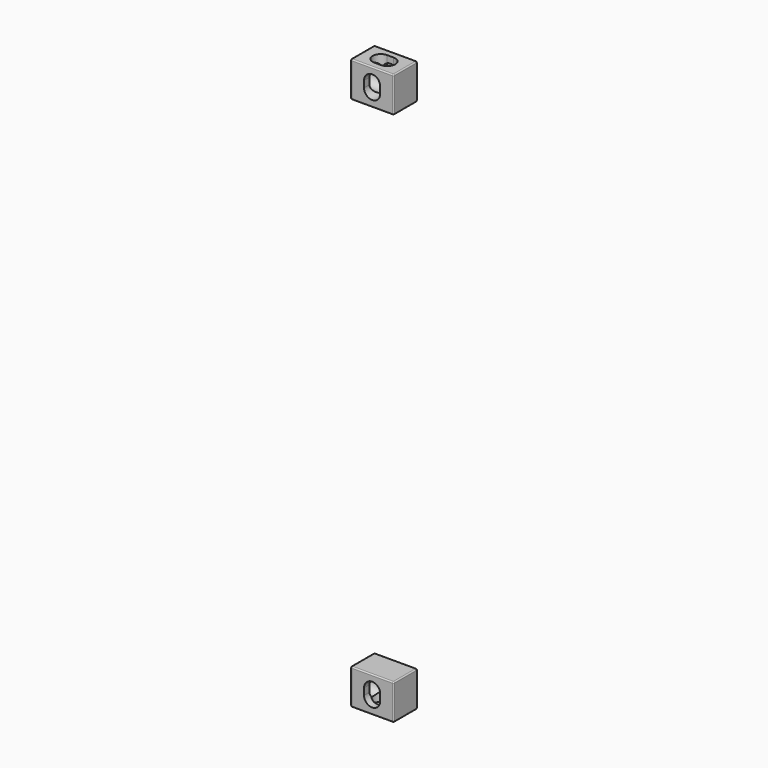
from build123d import *

# Parameters (mm, degrees)
F0_W          = 184
F0_H          = 127
F1_DEPTH      = 152
F3_DEPTH      = 122
F5_DEPTH      = 92
F7_DEPTH      = 78
F8_R          = 5
F9_R          = 5
F10_T1_DEPTH  = 159.5
F10_T3_DEPTH  = 142
F10_T5_DEPTH  = 191.5
F10_T7_DEPTH  = 117
F10_S11_W     = 5
F10_S11_H     = 5
F10_T12_DEPTH = 5
F10_S17_W     = 5
F10_S17_H     = 5
F10_T18_DEPTH = 5
F10_S23_W     = 5
F10_S23_H     = 5
F10_T24_DEPTH = 5
F10_S29_W     = 5
F10_S29_H     = 5
F10_T30_DEPTH = 5
F11_T1_DEPTH  = 117
F11_S5_W      = 5
F11_S5_H      = 5
F11_T6_DEPTH  = 5
F11_S11_W     = 5
F11_S11_H     = 5
F11_T12_DEPTH = 5


# Not quite as in the source:
# - a fillet or chamfer that OpenCascade refuses, or shapes differently, is made with other operations: its cross-section is extruded or revolved along the edge and cut away or added


with BuildPart() as f1:
    # F0 (on Top) → F1 (new body)
    with BuildSketch(Plane.XY):
        with Locations((-47.3488530219, 42.2096716464)):
            Rectangle(F0_W, F0_H)
    extrude(amount=F1_DEPTH)

    # F2 (on face) → F3 (cut)
    with BuildSketch(Plane.XZ.offset(21.2903283536)):
        with BuildLine():
            Line((-81.879962092, 90), (-81.879962092, 76))
            Line((-81.879962092, 76), (-81.879962092, 62))
            ThreePointArc((-81.879962092, 62), (-47.3488530219, 27.4688909298), (-12.8177439517, 62))
            Line((-12.8177439517, 62), (-12.8177439517, 76))
            Line((-12.8177439517, 76), (-12.8177439517, 90))
            ThreePointArc((-12.8177439517, 90), (-47.3488530219, 124.5311090702), (-81.879962092, 90))
        make_face()
    extrude(amount=-F3_DEPTH, mode=Mode.SUBTRACT)

    # F4 (on face) → F5 (cut)
    with BuildSketch(Plane(origin=(-139.3488530219, 0, 0), x_dir=(0, -1, 0), z_dir=(-1, 0, 0))):
        with BuildLine():
            Line((-76.7407790178, 90.0138813162), (-76.7407790178, 76.0138813162))
            Line((-76.7407790178, 76.0138813162), (-76.7407790178, 62.0138813162))
            ThreePointArc((-76.7407790178, 62.0138813162), (-42.2096699476, 27.482772246), (-7.6785608775, 62.0138813162))
            Line((-7.6785608775, 62.0138813162), (-7.6785608775, 76.0138813162))
            Line((-7.6785608775, 76.0138813162), (-7.6785608775, 90.0138813162))
            ThreePointArc((-7.6785608775, 90.0138813162), (-42.2096699476, 124.5449903863), (-76.7407790178, 90.0138813162))
        make_face()
    extrude(amount=-F5_DEPTH, mode=Mode.SUBTRACT)

    # F6 (on face) → F7 (cut)
    with BuildSketch(Plane.XY.offset(152)):
        with BuildLine():
            Line((-33.3898597658, 76.7718884866), (-47.3898597658, 76.7718884866))
            Line((-47.3898597658, 76.7718884866), (-61.3898597658, 76.7718884866))
            ThreePointArc((-61.3898597658, 76.7718884866), (-95.9209688359, 42.2407794164), (-61.3898597658, 7.7096703462))
            Line((-61.3898597658, 7.7096703462), (-47.3898597658, 7.7096703462))
            Line((-47.3898597658, 7.7096703462), (-33.3898597658, 7.7096703462))
            ThreePointArc((-33.3898597658, 7.7096703462), (1.1412493044, 42.2407794164), (-33.3898597658, 76.7718884866))
        make_face()
    extrude(amount=-F7_DEPTH, mode=Mode.SUBTRACT)

    # F8
    f8_edges = [f1.edges().sort_by_distance(p)[0] for p in [
        (-47.348853, -21.290328, 152),
    ]]
    fillet(f8_edges, radius=F8_R)

    # F9
    f9_edges = [f1.edges().sort_by_distance(p)[0] for p in [
        (-139.348853, -21.290328, 73.5),
        (-139.348853, 44.709672, 152),
        (44.651147, 44.709672, 152),
        (-47.348853, 105.709672, 152),
        (44.651147, -21.290328, 73.5),
        (-47.348853, -21.290328, 0),
    ]]
    fillet(f9_edges, radius=F9_R)

    # F10: fillet of radius 5 on 4 edges, made by hand

    # F10_s2 → F10_t1 (cut)
    with BuildSketch(Plane.XY.offset(-12.5)):
        with BuildLine():
            ThreePointArc((-134.3488530219, 105.7096716464), (-137.8843869278, 104.2452055523), (-139.3488530219, 100.7096716464))
            Line((-139.3488530219, 100.7096716464), (-139.3488530219, 105.7096716464))
            Line((-139.3488530219, 105.7096716464), (-134.3488530219, 105.7096716464))
        make_face()
    extrude(amount=F10_T1_DEPTH, mode=Mode.SUBTRACT)

    # F10_s4 → F10_t3 (cut)
    with BuildSketch(Plane.XY.offset(5)):
        with BuildLine():
            ThreePointArc((44.6511469781, 100.7096716464), (43.1866808841, 104.2452055523), (39.6511469781, 105.7096716464))
            Line((39.6511469781, 105.7096716464), (44.6511469781, 105.7096716464))
            Line((44.6511469781, 105.7096716464), (44.6511469781, 100.7096716464))
        make_face()
    extrude(amount=F10_T3_DEPTH, mode=Mode.SUBTRACT)

    # F10_s6 → F10_t5 (cut)
    with BuildSketch(Plane.YZ.offset(-151.8488530219)):
        with BuildLine():
            ThreePointArc((100.7096716464, 0), (104.2452055523, 1.4644660941), (105.7096716464, 5))
            Line((105.7096716464, 5), (105.7096716464, 0))
            Line((105.7096716464, 0), (100.7096716464, 0))
        make_face()
    extrude(amount=F10_T5_DEPTH, mode=Mode.SUBTRACT)

    # F10_s8 → F10_t7 (cut)
    with BuildSketch(Plane.XZ.offset(-100.7096716464)):
        with BuildLine():
            ThreePointArc((44.6511469781, 5), (43.1866808841, 1.4644660941), (39.6511469781, 0))
            Line((39.6511469781, 0), (44.6511469781, 0))
            Line((44.6511469781, 0), (44.6511469781, 5))
        make_face()
    extrude(amount=F10_T7_DEPTH, mode=Mode.SUBTRACT)


with BuildPart() as f10_tool10:
    # F10_s11 → F10_t12 (new body)
    with BuildSketch(Plane.YZ.offset(39.6511469781)):
        with Locations((-18.7903283536, 2.5)):
            Rectangle(F10_S11_W, F10_S11_H)
    extrude(amount=F10_T12_DEPTH)

    # F10_s13 → F10_t14 (revolve, cut)
    with BuildSketch(Plane(origin=(39.6511469781, -16.2903283536, 5), x_dir=(0, 0.7071067812, 0.7071067812), z_dir=(0, 0.7071067812, -0.7071067812))):
        with BuildLine():
            ThreePointArc((0, -5), (5, 0), (0, 5))
            Line((0, 5), (0, -5))
        make_face()
    revolve(axis=Axis((39.6511469781, -16.2903283536, 5), (1, 0, 0)), mode=Mode.SUBTRACT)


with BuildPart() as f1_1:
    add(f1.part)

    # F10_t9: cut F10_tool10
    add(f10_tool10.part, mode=Mode.SUBTRACT)


with BuildPart() as f10_tool16:
    # F10_s17 → F10_t18 (new body)
    with BuildSketch(Plane.YZ.offset(39.6511469781)):
        with Locations((103.2096716464, 149.5)):
            Rectangle(F10_S17_W, F10_S17_H)
    extrude(amount=F10_T18_DEPTH)

    # F10_s19 → F10_t20 (revolve, cut)
    with BuildSketch(Plane(origin=(39.6511469781, 100.7096716464, 147), x_dir=(0, -0.7071067812, -0.7071067812), z_dir=(0, -0.7071067812, 0.7071067812))):
        with BuildLine():
            ThreePointArc((0, -5), (5, 0), (0, 5))
            Line((0, 5), (0, -5))
        make_face()
    revolve(axis=Axis((39.6511469781, 100.7096716464, 147), (1, 0, 0)), mode=Mode.SUBTRACT)


with BuildPart() as f1_2:
    add(f1_1.part)

    # F10_t15: cut F10_tool16
    add(f10_tool16.part, mode=Mode.SUBTRACT)


with BuildPart() as f10_tool22:
    # F10_s23 → F10_t24 (new body)
    with BuildSketch(Plane.XZ.offset(-100.7096716464)):
        with Locations((-136.8488530219, 149.5)):
            Rectangle(F10_S23_W, F10_S23_H)
    extrude(amount=-F10_T24_DEPTH)

    # F10_s25 → F10_t26 (revolve, cut)
    with BuildSketch(Plane(origin=(-134.3488530219, 100.7096716464, 147), x_dir=(0.7071067812, 0, -0.7071067812), z_dir=(0.7071067812, 0, 0.7071067812))):
        with BuildLine():
            ThreePointArc((0, -5), (5, 0), (0, 5))
            Line((0, 5), (0, -5))
        make_face()
    revolve(axis=Axis((-134.3488530219, 100.7096716464, 147), (0, 1, 0)), mode=Mode.SUBTRACT)


with BuildPart() as f1_3:
    add(f1_2.part)

    # F10_t21: cut F10_tool22
    add(f10_tool22.part, mode=Mode.SUBTRACT)


with BuildPart() as f10_tool28:
    # F10_s29 → F10_t30 (new body)
    with BuildSketch(Plane.YZ.offset(39.6511469781)):
        with Locations((103.2096716464, 2.5)):
            Rectangle(F10_S29_W, F10_S29_H)
    extrude(amount=F10_T30_DEPTH)

    # F10_s31 → F10_t32 (revolve, cut)
    with BuildSketch(Plane(origin=(39.6511469781, 100.7096716464, 5), x_dir=(0, -0.7071067812, 0.7071067812), z_dir=(0, 0.7071067812, 0.7071067812))):
        with BuildLine():
            ThreePointArc((0, -5), (5, 0), (0, 5))
            Line((0, 5), (0, -5))
        make_face()
    revolve(axis=Axis((39.6511469781, 100.7096716464, 5), (1, 0, 0)), mode=Mode.SUBTRACT)


with BuildPart() as f1_4:
    add(f1_3.part)

    # F10_t27: cut F10_tool28
    add(f10_tool28.part, mode=Mode.SUBTRACT)

    # F11: fillet of radius 5 on 1 edges, made by hand

    # F11_s2 → F11_t1 (cut)
    with BuildSketch(Plane.XZ.offset(-100.7096716464)):
        with BuildLine():
            ThreePointArc((-134.3488530219, 0), (-137.8843869278, 1.4644660941), (-139.3488530219, 5))
            Line((-139.3488530219, 5), (-139.3488530219, 0))
            Line((-139.3488530219, 0), (-134.3488530219, 0))
        make_face()
    extrude(amount=F11_T1_DEPTH, mode=Mode.SUBTRACT)


with BuildPart() as f11_tool4:
    # F11_s5 → F11_t6 (new body)
    with BuildSketch(Plane.XY.offset(5)):
        with Locations((-136.8488530219, 103.2096716464)):
            Rectangle(F11_S5_W, F11_S5_H)
    extrude(amount=-F11_T6_DEPTH)

    # F11_s7 → F11_t8 (revolve, cut)
    with BuildSketch(Plane(origin=(-134.3488530219, 100.7096716464, 5), x_dir=(0.7071067812, -0.7071067812, 0), z_dir=(0.7071067812, 0.7071067812, 0))):
        with BuildLine():
            ThreePointArc((0, -5), (5, 0), (0, 5))
            Line((0, 5), (0, -5))
        make_face()
    revolve(axis=Axis((-134.3488530219, 100.7096716464, 5), (0, 0, -1)), mode=Mode.SUBTRACT)


with BuildPart() as f1_5:
    add(f1_4.part)

    # F11_t3: cut F11_tool4
    add(f11_tool4.part, mode=Mode.SUBTRACT)


with BuildPart() as f11_tool10:
    # F11_s11 → F11_t12 (new body)
    with BuildSketch(Plane.XY.offset(5)):
        with Locations((-136.8488530219, -18.7903283536)):
            Rectangle(F11_S11_W, F11_S11_H)
    extrude(amount=-F11_T12_DEPTH)

    # F11_s13 → F11_t14 (revolve, cut)
    with BuildSketch(Plane(origin=(-134.3488530219, -16.2903283536, 5), x_dir=(0.7071067812, 0.7071067812, 0), z_dir=(-0.7071067812, 0.7071067812, 0))):
        with BuildLine():
            ThreePointArc((0, -5), (5, 0), (0, 5))
            Line((0, 5), (0, -5))
        make_face()
    revolve(axis=Axis((-134.3488530219, -16.2903283536, 5), (0, 0, -1)), mode=Mode.SUBTRACT)


with BuildPart() as f1_6:
    add(f1_5.part)

    # F11_t9: cut F11_tool10
    add(f11_tool10.part, mode=Mode.SUBTRACT)


with BuildPart() as f13_1:
    # F13: instance of F1
    add(f1_6.part.mirror(Plane.XY.offset(-1067)))


solid = Compound([f1_6.part, f13_1.part])
